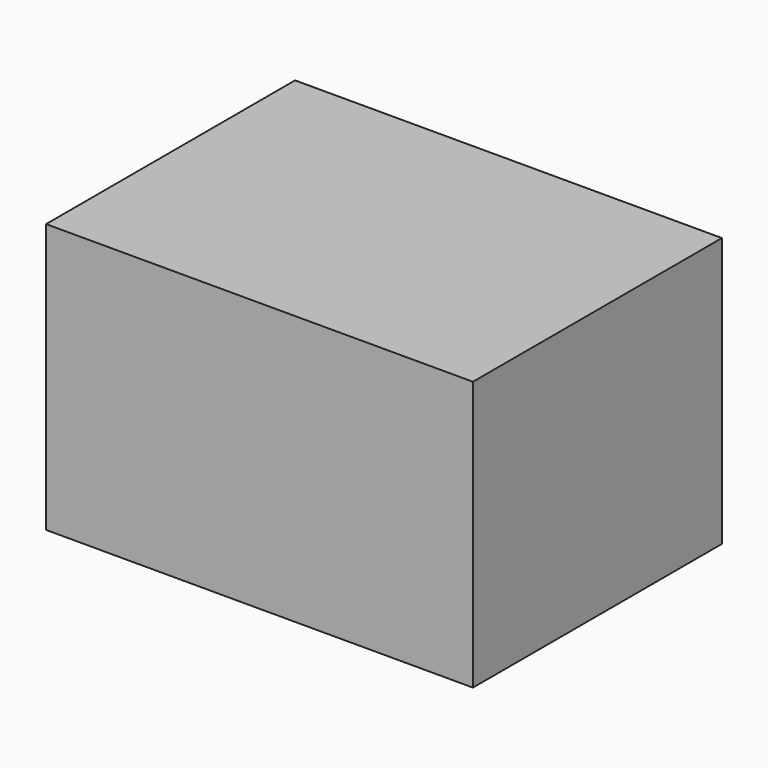
from build123d import *

# Parameters (mm, degrees)
F0_W     = 90.9976512194
F0_H     = 66.3465689868
F1_DEPTH = 57.404


# Not quite as in the source:
# - the program builds the solid bodies; features that only make, move or delete a surface that nothing else refers to are left out


with BuildPart() as f1:
    # F0 (on Top) → F1 (new body)
    with BuildSketch(Plane.XY):
        with Locations((-9.687051177, -4.9651348963)):
            Rectangle(F0_W, F0_H)
    extrude(amount=F1_DEPTH)


solid = f1.part
